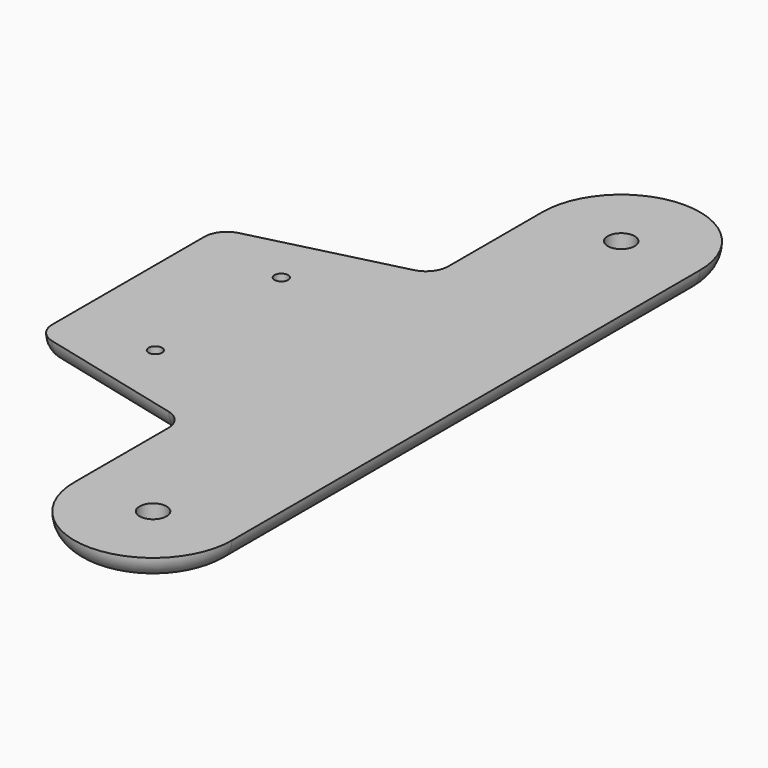
from build123d import *

# Parameters (mm, degrees)
F0_R     = 1.5
F0_R_2   = 3
F1_DEPTH = 5
F2_R     = 4.99999


# Not quite as in the source:
# - a fillet or chamfer is up to 0.001 mm smaller than in the source, because OpenCascade refuses the exact size


with BuildPart() as f1:
    # F0 (on Top) → F1 (new body)
    with BuildSketch(Plane.XY):
        with BuildLine():
            Line((17.5, -65), (17.5, 65))
            ThreePointArc((17.5, 65), (0, 82.5), (-17.5, 65))
            Line((-17.5, 65), (-17.5, 38.903882032))
            ThreePointArc((-17.5, 38.903882032), (-18.5589728099, 35.826820985), (-21.2873218748, 34.0531695313))
            Line((-21.2873218748, 34.0531695313), (-53.7126781252, 25.9468304687))
            ThreePointArc((-53.7126781252, 25.9468304687), (-56.4410271901, 24.173179015), (-57.5, 21.096117968))
            Line((-57.5, 21.096117968), (-57.5, -21.096117968))
            ThreePointArc((-57.5, -21.096117968), (-56.4410271901, -24.173179015), (-53.7126781252, -25.9468304687))
            Line((-53.7126781252, -25.9468304687), (-21.2873218748, -34.0531695313))
            ThreePointArc((-21.2873218748, -34.0531695313), (-18.5589728099, -35.826820985), (-17.5, -38.903882032))
            Line((-17.5, -38.903882032), (-17.5, -65))
            ThreePointArc((-17.5, -65), (0, -82.5), (17.5, -65))
        make_face()
        with Locations((-37.5, -17.5)):
            Circle(F0_R, mode=Mode.SUBTRACT)
        with Locations((0, -65)):
            Circle(F0_R_2, mode=Mode.SUBTRACT)
        with Locations((-37.5, 17.5)):
            Circle(F0_R, mode=Mode.SUBTRACT)
        with Locations((0, 65)):
            Circle(F0_R_2, mode=Mode.SUBTRACT)
    extrude(amount=F1_DEPTH)

    # F2 (radius 5 in the source; OpenCascade refuses exactly that, so slightly less here)
    f2_edges = [f1.edges().sort_by_distance(p)[0] for p in [
        (17.5, 0, 0),
    ]]
    fillet(f2_edges, radius=F2_R)


solid = f1.part
